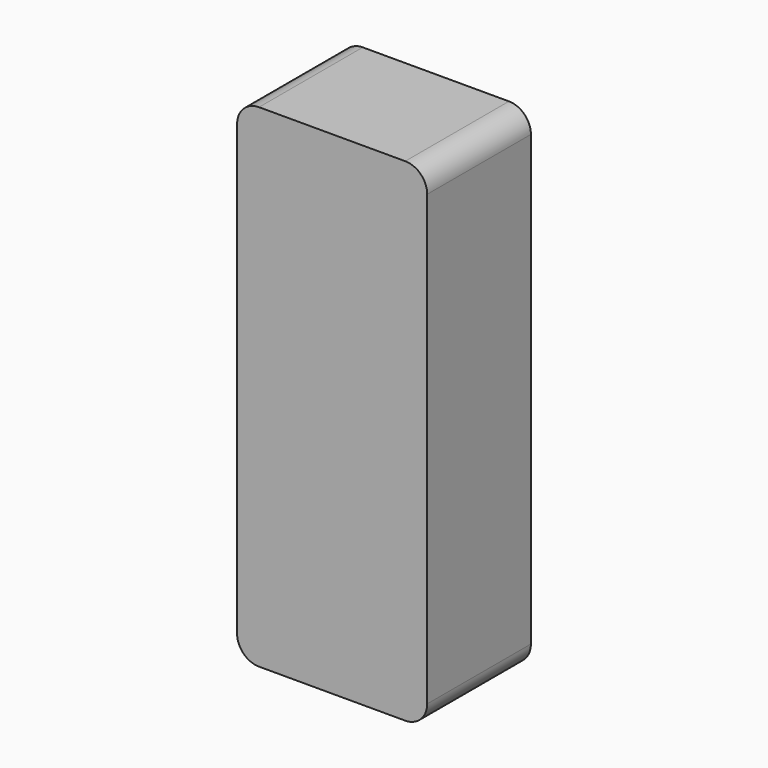
from build123d import *

# Parameters (mm, degrees)
F0_W        = 44
F0_H        = 30
F1_DEPTH    = 114
F2_W        = 35
F2_H        = 105
F3_DEPTH    = 26
F4_R        = 5.08
F5_R        = 2.4528409794
F6_W        = 22.4547982216
F6_H        = 9.9273854867
F7_DEPTH    = 5.08
F8_T1_DEPTH = 22.4547982216


# Not quite as in the source:
# - a fillet or chamfer that OpenCascade refuses, or shapes differently, is made with other operations: its cross-section is extruded or revolved along the edge and cut away or added


with BuildPart() as f1:
    # F0 (on Top) → F1 (new body)
    with BuildSketch(Plane.XY):
        Rectangle(F0_W, F0_H)
    extrude(amount=F1_DEPTH)

    # F2 (on face) → F3 (cut)
    with BuildSketch(Plane(origin=(0, 15, 0), x_dir=(-1, 0, 0), z_dir=(0, 1, 0))):
        with Locations((0.5, 57.5)):
            Rectangle(F2_W, F2_H)
    extrude(amount=-F3_DEPTH, mode=Mode.SUBTRACT)

    # F4
    f4_edges = [f1.edges().sort_by_distance(p)[0] for p in [
        (22, 0, 0),
        (-22, 0, 0),
        (-22, 0, 114),
        (22, 0, 114),
    ]]
    fillet(f4_edges, radius=F4_R)

    # F5
    f5_edges = [f1.edges().sort_by_distance(p)[0] for p in [
        (17, 2, 110),
        (-18, 2, 110),
        (17, 2, 5),
        (-18, 2, 5),
    ]]
    fillet(f5_edges, radius=F5_R)

    # F6 (on face) → F7 (cut)
    with BuildSketch(Plane(origin=(0, 0, 0), x_dir=(1, 0, 0), z_dir=(0, 0, -1))):
        with Locations((0, 9.9273854867)):
            Rectangle(F6_W, F6_H)
    extrude(amount=-F7_DEPTH, mode=Mode.SUBTRACT)

    # F8: fillet of radius 5.08 on 1 edges, made by hand

    # F8_s2 → F8_t1 (join)
    with BuildSketch(Plane.YZ.offset(-11.2273991108)):
        with BuildLine():
            ThreePointArc((-14.89107823, 0.1410866555), (-13.8014493024, 3.2848644314), (-11, 5.08))
            Line((-11, 5.08), (-14.89107823, 5.08))
            Line((-14.89107823, 5.08), (-14.89107823, 0.1410866555))
        make_face()
    extrude(amount=F8_T1_DEPTH)


solid = f1.part
